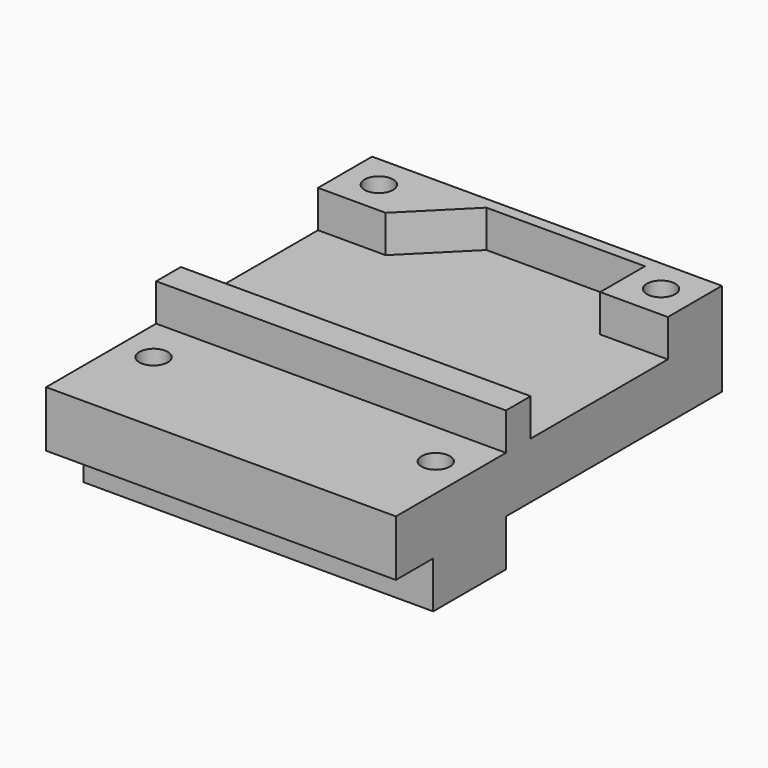
from build123d import *

# Parameters (mm, degrees)
F0_W           = 30
F0_H           = 23.15
F0_H_2         = 6.8
F0_R           = 1.3
F0_H_3         = 4
F0_H_4         = 1
F1_DEPTH       = 12
F2_W           = 5.8
F2_H           = 5.8
F3_DEPTH       = 3.2
F4_DEPTH       = 4
F5_D           = 2.4384
F5_DEPTH       = 10
F5_CBORE_D     = 4.7625
F5_CBORE_DEPTH = 2.1844
F5_TIP         = 0.7325692667
F6_D           = 2.4384
F6_DEPTH       = 20
F6_START       = 4
F6_TIP         = 0.7325692667
F7_DEPTH       = 6


# Not quite as in the source:
# - a feature names something its author has since deleted; it is built from what else it names


with BuildPart() as f1:
    # F0 (on Top) → F1 (new body)
    with BuildSketch(Plane.XY):
        with Locations((0, 23.375)):
            Rectangle(F0_W, F0_H)
        Polygon((-10.7251846715, 34.43125), (-9.350369343, 32.05), (-10.7251846715, 29.66875), (-13.4748153285, 29.66875), (-14.849630657, 32.05), (-13.4748153285, 34.43125), align=None, mode=Mode.SUBTRACT)
        Polygon((10.7251846715, 29.66875), (9.350369343, 32.05), (10.7251846715, 34.43125), (13.4748153285, 34.43125), (14.849630657, 32.05), (13.4748153285, 29.66875), align=None, mode=Mode.SUBTRACT)
        with Locations((0, 7.4)):
            Rectangle(F0_W, F0_H_2)
        with Locations((-12.1, 7.9)):
            Circle(F0_R, mode=Mode.SUBTRACT)
        with Locations((12.1, 7.9)):
            Circle(F0_R, mode=Mode.SUBTRACT)
        with Locations((0, 2)):
            Rectangle(F0_W, F0_H_3)
        with Locations((0, 11.3)):
            Rectangle(F0_W, F0_H_4)
        Polygon((-10.7251846715, 29.66875), (-9.350369343, 32.05), (-10.7251846715, 34.43125), (-13.4748153285, 34.43125), (-14.849630657, 32.05), (-13.4748153285, 29.66875), align=None)
        with Locations((-12.1, 32.05)):
            Circle(F0_R, mode=Mode.SUBTRACT)
        Polygon((10.7251846715, 34.43125), (9.350369343, 32.05), (10.7251846715, 29.66875), (13.4748153285, 29.66875), (14.849630657, 32.05), (13.4748153285, 34.43125), align=None)
        with Locations((12.1, 32.05)):
            Circle(F0_R, mode=Mode.SUBTRACT)
        with Locations((-12.1, 32.05)):
            Circle(F0_R)
        with Locations((12.1, 32.05)):
            Circle(F0_R)
        with Locations((12.1, 7.9)):
            Circle(F0_R)
        with Locations((-12.1, 7.9)):
            Circle(F0_R)
    extrude(amount=F1_DEPTH)

    # F2 (on face) → F3 (cut)
    with BuildSketch(Plane.XY.offset(12)):
        with Locations((-12.1, 7.9)):
            Rectangle(F2_W, F2_H)
        Polygon((9.2, 5), (9.2, 10.8), (-9.2, 10.8), (-9.2, 5), (-15, 5), (-15, 0), (15, 0), (15, 5), align=None)
        with Locations((12.1, 7.9)):
            Rectangle(F2_W, F2_H)
        Polygon((9.2, 10.8), (15, 10.8), (15, 11.8), (-15, 11.8), (-15, 10.8), (-9.2, 10.8), align=None)
        Polygon((-3.4, 14.45), (9.2, 14.45), (9.2, 20.25), (15, 20.25), (15, 29.15), (9.2, 29.15), (9.2, 33.95), (-4.4, 33.95), (-9.2, 29.15), (-13.65, 24.7), (-9.2, 20.25), align=None)
        Polygon((-15, 23.35), (-15, 20.25), (-9.2, 20.25), (-13.65, 24.7), align=None)
        Polygon((-15, 26.05), (-13.65, 24.7), (-9.2, 29.15), (-15, 29.15), align=None)
        Polygon((-15, 26.05), (-15, 23.35), (-13.65, 24.7), align=None)
        Polygon((-9.2, 14.45), (-3.4, 14.45), (-9.2, 20.25), align=None)
        with Locations((-12.1, 17.35)):
            Rectangle(F2_W, F2_H)
        with Locations((12.1, 17.35)):
            Rectangle(F2_W, F2_H)
    extrude(amount=-F3_DEPTH, mode=Mode.SUBTRACT)

    # F0 (on Top) → F4 (cut)
    with BuildSketch(Plane.XY):
        with Locations((0, 23.375)):
            Rectangle(F0_W, F0_H)
        Polygon((-10.7251846715, 34.43125), (-9.350369343, 32.05), (-10.7251846715, 29.66875), (-13.4748153285, 29.66875), (-14.849630657, 32.05), (-13.4748153285, 34.43125), align=None, mode=Mode.SUBTRACT)
        Polygon((10.7251846715, 29.66875), (9.350369343, 32.05), (10.7251846715, 34.43125), (13.4748153285, 34.43125), (14.849630657, 32.05), (13.4748153285, 29.66875), align=None, mode=Mode.SUBTRACT)
        with Locations((0, 2)):
            Rectangle(F0_W, F0_H_3)
        Polygon((-10.7251846715, 29.66875), (-9.350369343, 32.05), (-10.7251846715, 34.43125), (-13.4748153285, 34.43125), (-14.849630657, 32.05), (-13.4748153285, 29.66875), align=None)
        with Locations((-12.1, 32.05)):
            Circle(F0_R, mode=Mode.SUBTRACT)
        Polygon((10.7251846715, 34.43125), (9.350369343, 32.05), (10.7251846715, 29.66875), (13.4748153285, 29.66875), (14.849630657, 32.05), (13.4748153285, 34.43125), align=None)
        with Locations((12.1, 32.05)):
            Circle(F0_R, mode=Mode.SUBTRACT)
        with Locations((-12.1, 32.05)):
            Circle(F0_R)
        with Locations((12.1, 32.05)):
            Circle(F0_R)
    extrude(amount=F4_DEPTH, mode=Mode.SUBTRACT)

    # F5
    with Locations(Plane(origin=(0, 0, 0), x_dir=(1, 0, 0), z_dir=(0, 0, -1))):
        with Locations((-12.1, -7.9), (12.1, -7.9)):
            CounterBoreHole(F5_D / 2, F5_CBORE_D / 2, F5_CBORE_DEPTH, depth=F5_DEPTH)
            with Locations((0, 0, -(F5_DEPTH + F5_TIP / 2))):  # 118° drill point
                Cone(0, F5_D / 2, F5_TIP, mode=Mode.SUBTRACT)

    # F6
    # its depths count from where the whole tool has entered the part; down to there all is cleared
    with Locations(Plane(origin=(0, 0, 0), x_dir=(1, 0, 0), z_dir=(0, 0, -1)).offset(-F6_START)):
        with Locations((-12.1, -32.05), (12.1, -32.05)):
            Hole(F6_D / 2, depth=F6_DEPTH)
            with Locations((0, 0, -(F6_DEPTH + F6_TIP / 2))):  # 118° drill point
                Cone(0, F6_D / 2, F6_TIP, mode=Mode.SUBTRACT)

    # F0 (on Top) → F7 (cut)
    with BuildSketch(Plane.XY):
        Polygon((-10.7251846715, 29.66875), (-9.350369343, 32.05), (-10.7251846715, 34.43125), (-13.4748153285, 34.43125), (-14.849630657, 32.05), (-13.4748153285, 29.66875), align=None)
        with Locations((-12.1, 32.05)):
            Circle(F0_R, mode=Mode.SUBTRACT)
        Polygon((10.7251846715, 34.43125), (9.350369343, 32.05), (10.7251846715, 29.66875), (13.4748153285, 29.66875), (14.849630657, 32.05), (13.4748153285, 34.43125), align=None)
        with Locations((12.1, 32.05)):
            Circle(F0_R, mode=Mode.SUBTRACT)
        with Locations((12.1, 32.05)):
            Circle(F0_R)
        with Locations((-12.1, 32.05)):
            Circle(F0_R)
    extrude(amount=F7_DEPTH, mode=Mode.SUBTRACT)


solid = f1.part
